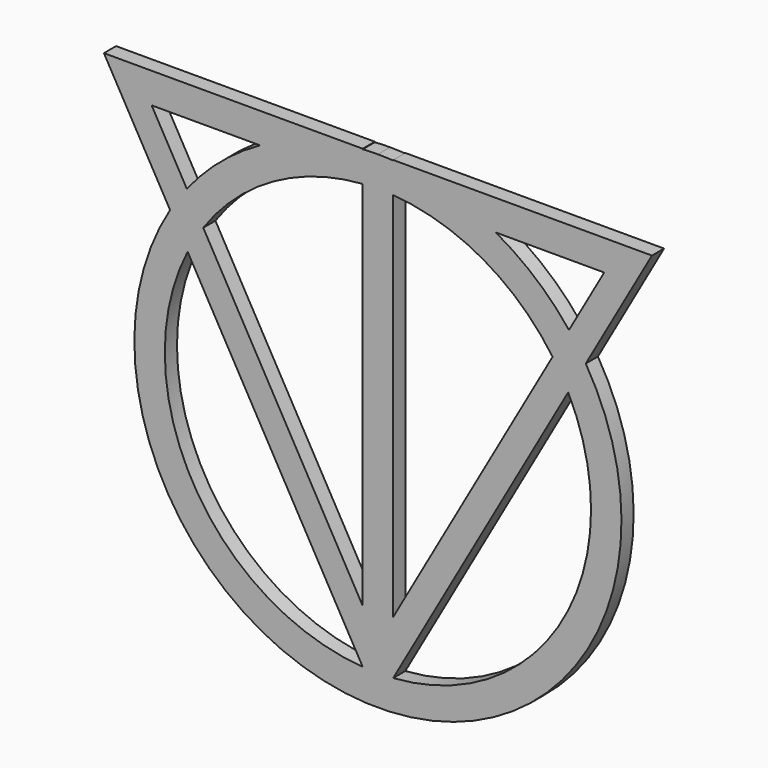
from build123d import *

# Parameters (mm, degrees)
F1_DEPTH = 3.175


# Not quite as in the source:
# - a length typed as a fraction of an inch, garbled in the dataset ("3 / 203.2 mm" for 3/8 in), is restored


with BuildPart() as f1:
    # F0 (on Front) → F1 (new body)
    with BuildSketch(Plane.XZ):
        with BuildLine():
            ThreePointArc((-43.3524121445, 26.4803391454), (-44.3048599399, -24.8539611673), (0, -50.8))
            ThreePointArc((0, -50.8), (44.3048599399, -24.8539611673), (43.3524121445, 26.4803391454))
            Line((43.3524121445, 26.4803391454), (57.15, 50.8))
            Line((57.15, 50.8), (50.8, 50.8))
            Line((50.8, 50.8), (3.175, 50.8))
            Line((3.175, 50.8), (3.175, 50.700684167))
            ThreePointArc((3.175, 50.700684167), (1.5882764743, 50.7751649711), (0, 50.8))
            ThreePointArc((0, 50.8), (-1.5882764743, 50.7751649711), (-3.175, 50.700684167))
            Line((-3.175, 50.700684167), (-3.175, 50.8))
            Line((-3.175, 50.8), (-50.8, 50.8))
            Line((-50.8, 50.8), (-57.15, 50.8))
            Line((-57.15, 50.8), (-43.3524121445, 26.4803391454))
        make_face()
        with BuildLine():
            Line((-39.6867141727, 20.0191712658), (-3.175, -44.336462139))
            ThreePointArc((-3.175, -44.336462139), (-38.6612664458, -21.9341965162), (-39.6867141727, 20.0191712658))
        make_face(mode=Mode.SUBTRACT)
        with BuildLine():
            ThreePointArc((39.6867141727, 20.0191712658), (38.6612664458, -21.9341965162), (3.175, -44.336462139))
            Line((3.175, -44.336462139), (39.6867141727, 20.0191712658))
        make_face(mode=Mode.SUBTRACT)
        with BuildLine():
            ThreePointArc((-36.429171038, 25.4699430208), (-21.9341965162, 38.6612664458), (-3.175, 44.336462139))
            Line((-3.175, 44.336462139), (-3.175, -33.1439371814))
            Line((-3.175, -33.1439371814), (-36.429171038, 25.4699430208))
        make_face(mode=Mode.SUBTRACT)
        with BuildLine():
            Line((-47.1973723398, 44.45), (-24.5934442484, 44.45))
            ThreePointArc((-24.5934442484, 44.45), (-32.8665744068, 38.7353622258), (-39.8520903437, 31.5031886519))
            Line((-39.8520903437, 31.5031886519), (-47.1973723398, 44.45))
        make_face(mode=Mode.SUBTRACT)
        with BuildLine():
            Line((3.175, -33.1439371814), (3.175, 44.336462139))
            ThreePointArc((3.175, 44.336462139), (21.9341965162, 38.6612664458), (36.429171038, 25.4699430208))
            Line((36.429171038, 25.4699430208), (3.175, -33.1439371814))
        make_face(mode=Mode.SUBTRACT)
        with BuildLine():
            ThreePointArc((39.8520903437, 31.5031886519), (32.8665744068, 38.7353622258), (24.5934442484, 44.45))
            Line((24.5934442484, 44.45), (47.1973723398, 44.45))
            Line((47.1973723398, 44.45), (39.8520903437, 31.5031886519))
        make_face(mode=Mode.SUBTRACT)
    extrude(amount=F1_DEPTH)


solid = f1.part
